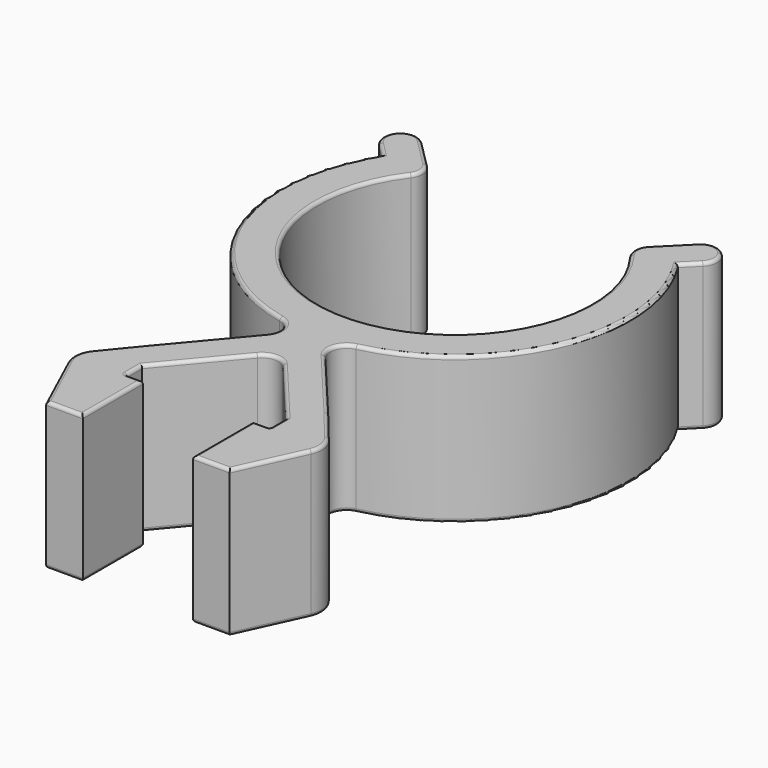
from build123d import *

# Parameters (mm, degrees)
F1_DEPTH      = 8.8
F2_R          = 0.99999
F3_R          = 0.1
F4_R          = 1
F6_T3_DEPTH   = 5.9978588629
F6_T7_ANGLE   = 100
F6_T10_DEPTH  = 1.6
F6_T14_DEPTH  = 5.9978588629
F6_T18_ANGLE  = 90
F6_T21_DEPTH  = 1.6
F6_T25_DEPTH  = 1.4
F6_T28_ANGLE  = 90
F6_T31_DEPTH  = 5.5
F6_T34_DEPTH  = 1.4
F6_T37_DEPTH  = 3.2
F6_T40_DEPTH  = 5.5
F6_T43_DEPTH  = 6.2023355211
F6_T46_DEPTH  = 3.2
F6_T49_DEPTH  = 3.9268834236
F6_T52_DEPTH  = 6.2023355211
F6_T55_DEPTH  = 5.8449118324
F6_T58_DEPTH  = 3.9268834236
F6_T61_ANGLE  = 117.3981887598
F6_T64_DEPTH  = 5.8449118324
F6_T67_ANGLE  = 112.5286263579
F6_T71_ANGLE  = 117.3981887598
F6_T74_DEPTH  = 1.680236188
F6_S75_R      = 10.5
F6_T76_DEPTH  = 2
F6_T79_ANGLE  = 112.5286263579
F6_T83_ANGLE  = 83.5571716204
F6_T86_DEPTH  = 1.680236188
F6_S87_R      = 10.5
F6_T88_DEPTH  = 2
F6_T91_ANGLE  = 0.0001002781
F6_T94_ANGLE  = 83.5571716204
F6_T97_ANGLE  = 96.4427281016
F6_T100_ANGLE = 0.0001002781
F6_T103_DEPTH = 2.3183400779
F6_T106_ANGLE = 96.4427281016
F6_T109_ANGLE = 81.9369478746
F6_T112_DEPTH = 2.3183400779
F6_T115_ANGLE = 253.8738957492
F6_T118_ANGLE = 81.9369478746
F6_T121_DEPTH = 5.9978588629
F6_T125_ANGLE = 100
F6_T128_DEPTH = 1.6
F6_T132_DEPTH = 5.9978588629
F6_T136_ANGLE = 90
F6_T139_DEPTH = 1.6
F6_T143_DEPTH = 1.4
F6_T146_ANGLE = 90
F6_T149_DEPTH = 5.5
F6_T152_DEPTH = 1.4
F6_T155_DEPTH = 3.2
F6_T158_DEPTH = 5.5
F6_T161_DEPTH = 6.2023355211
F6_T164_DEPTH = 3.2
F6_T167_DEPTH = 3.9268834236
F6_T170_DEPTH = 6.2023355211
F6_T173_DEPTH = 5.8449118324
F6_T176_DEPTH = 3.9268834236
F6_T179_ANGLE = 117.3981887598
F6_T182_DEPTH = 5.8449118324
F6_T185_ANGLE = 112.5286263579
F6_T189_ANGLE = 117.3981887598
F6_T192_DEPTH = 1.680236188
F6_S193_R     = 10.5
F6_T194_DEPTH = 2
F6_T197_ANGLE = 112.5286263579
F6_T201_ANGLE = 83.5571716204
F6_T204_DEPTH = 1.680236188
F6_S205_R     = 10.5
F6_T206_DEPTH = 2
F6_T209_ANGLE = 0.0001002781
F6_T212_ANGLE = 83.5571716204
F6_T215_ANGLE = 96.4427281016
F6_T218_ANGLE = 0.0001002781
F6_T221_DEPTH = 2.3183400779
F6_T224_ANGLE = 96.4427281016
F6_T227_ANGLE = 81.9369478746
F6_T230_DEPTH = 2.3183400779
F6_T233_ANGLE = 253.8738957492
F6_T236_ANGLE = 81.9369478746
F6_T240_DEPTH = 5.9978588629
F6_T244_DEPTH = 1.6
F6_T250_DEPTH = 5.9978588629
F6_T254_DEPTH = 1.6
F6_T260_ANGLE = 112.5286263579
F6_T264_DEPTH = 1.680236188
F6_S265_R     = 10.5
F6_T266_DEPTH = 2
F6_T271_ANGLE = 112.5286263579
F6_T275_DEPTH = 1.680236188
F6_S276_R     = 10.5
F6_T277_DEPTH = 2
F6_T282_DEPTH = 5.9978588629
F6_T286_DEPTH = 1.6
F6_T292_DEPTH = 5.9978588629
F6_T296_DEPTH = 1.6
F6_T302_ANGLE = 112.5286263579
F6_T306_DEPTH = 1.680236188
F6_S307_R     = 10.5
F6_T308_DEPTH = 2
F6_T313_ANGLE = 112.5286263579
F6_T317_DEPTH = 1.680236188
F6_S318_R     = 10.5
F6_T319_DEPTH = 2
F7_T1_DEPTH   = 8.8000000003
F7_T4_ANGLE   = 63.917692294
F7_T6_ANGLE   = 63.917692294
F7_T8_ANGLE   = 63.917692294
F7_T10_ANGLE  = 63.917692294


# Not quite as in the source:
# - a fillet or chamfer that OpenCascade refuses, or shapes differently, is made with other operations: its cross-section is extruded or revolved along the edge and cut away or added
# - a fillet or chamfer is up to 0.001 mm smaller than in the source, because OpenCascade refuses the exact size
# - a feature of the source that left no trace in its solid (it failed there, or was rolled back) is left out


with BuildPart() as f1:
    # F0 (on Top) → F1 (new body)
    with BuildSketch(Plane.XY):
        with BuildLine():
            ThreePointArc((6, 5.589275445), (0, -8.2), (-6, 5.589275445))
            Line((-6, 5.589275445), (-9.0418110175, 8.6310864625))
            ThreePointArc((-9.0418110175, 8.6310864625), (-9.706736329, 7.8758662913), (-10.3087630343, 7.0696113545))
            Line((-10.3087630343, 7.0696113545), (-8.8654004375, 5.6262487577))
            ThreePointArc((-8.8654004375, 5.6262487577), (-9.338258559, -4.8007215171), (-0.5833668689, -10.4837819081))
            Line((-0.5833668689, -10.4837819081), (-5.5, -16.3431971055))
            Line((-5.5, -16.3431971055), (-7.669290062, -18.9960654825))
            Line((-7.669290062, -18.9960654825), (-5.5, -23.7245404482))
            Line((-5.5, -23.7245404482), (-3.3, -23.7245404482))
            Line((-3.3, -23.7245404482), (-3.3, -19.2245404482))
            Line((-3.3, -19.2245404482), (-4.3, -19.2245404482))
            Line((-4.3, -19.2245404482), (-4.3, -18.0245404482))
            Line((-4.3, -18.0245404482), (0, -12.9))
            Line((0, -12.9), (4.3, -18.0245404482))
            Line((4.3, -18.0245404482), (4.3, -19.2245404482))
            Line((4.3, -19.2245404482), (3.3, -19.2245404482))
            Line((3.3, -19.2245404482), (3.3, -23.7245404482))
            Line((3.3, -23.7245404482), (5.5, -23.7245404482))
            Line((5.5, -23.7245404482), (7.669290062, -18.9960654825))
            Line((7.669290062, -18.9960654825), (5.5, -16.3431971055))
            Line((5.5, -16.3431971055), (1.5320888862, -11.6144247806))
            Line((1.5320888862, -11.6144247806), (0.5833668689, -10.4837819081))
            ThreePointArc((0.5833668689, -10.4837819081), (9.338258559, -4.8007215171), (8.8654004375, 5.6262487577))
            Line((8.8654004375, 5.6262487577), (10.3087630343, 7.0696113545))
            ThreePointArc((10.3087630343, 7.0696113545), (9.706736329, 7.8758662913), (9.0418110175, 8.6310864625))
            Line((9.0418110175, 8.6310864625), (6, 5.589275445))
        make_face()
    extrude(amount=F1_DEPTH)

    # F2 (radius 1 in the source; OpenCascade refuses exactly that, so slightly less here)
    f2_edges = [f1.edges().sort_by_distance(p)[0] for p in [
        (6, 5.589275, 4.4),
        (-6, 5.589275, 4.4),
        (-9.041811, 8.631086, 4.4),
        (9.041811, 8.631086, 4.4),
        (10.308763, 7.069611, 4.4),
        (-10.308763, 7.069611, 4.4),
        (0.583367, -10.483782, 4.4),
        (-0.583367, -10.483782, 4.4),
    ]]
    fillet(f2_edges, radius=F2_R)

    # F3
    f3_edges = [f1.edges().sort_by_distance(p)[0] for p in [
        (-4.3, -19.22454, 4.4),
        (4.3, -19.22454, 4.4),
    ]]
    fillet(f3_edges, radius=F3_R)

    # F4
    f4_edges = [f1.edges().sort_by_distance(p)[0] for p in [
        (0, -12.9, 4.4),
    ]]
    fillet(f4_edges, radius=F4_R)

    # F6: fillet of radius 0.2 on 72 edges, made by hand


with BuildPart() as f6_tool1:
    # F6_s2 → F6_t3 (new body)
    with BuildSketch(Plane(origin=(7.11805445, -8.4829669631, 0), x_dir=(0, 0, 1), z_dir=(0.6427876097, -0.7660444431, 0))):
        with BuildLine():
            ThreePointArc((8.6, 8.291960165), (8.7414213562, 8.2333815212), (8.8, 8.091960165))
            Line((8.8, 8.091960165), (8.8, 8.291960165))
            Line((8.8, 8.291960165), (8.6, 8.291960165))
        make_face()
    extrude(amount=F6_T3_DEPTH)

    split(bisect_by=Plane.YZ.offset(4.3), keep=Keep.BOTTOM)


with BuildPart() as f6_tool5:
    # F6_s6 → F6_t7 (revolve)
    with BuildSketch(Plane(origin=(7.11805445, -8.4829669631, 0), x_dir=(0, 0, 1), z_dir=(0.6427876097, -0.7660444431, 0))):
        with BuildLine():
            ThreePointArc((8.6, 8.291960165), (8.7414213562, 8.2333815212), (8.8, 8.091960165))
            Line((8.8, 8.091960165), (8.8, 8.291960165))
            Line((8.8, 8.291960165), (8.6, 8.291960165))
        make_face()
    revolve(axis=Axis((0, -14.4557238269, 8.8), (0, 0, 1)), revolution_arc=F6_T7_ANGLE)


with BuildPart() as f6_tool8:
    # F6_s9 → F6_t10 (new body)
    with BuildSketch(Plane.XZ.offset(17.5245404482)):
        with BuildLine():
            ThreePointArc((4.3, 8.6), (4.3585786438, 8.7414213562), (4.5, 8.8))
            Line((4.5, 8.8), (4.3, 8.8))
            Line((4.3, 8.8), (4.3, 8.6))
        make_face()
    extrude(amount=F6_T10_DEPTH)

    split(bisect_by=Plane(origin=(-6.3520100069, -5.329969254, 0), x_dir=(0, 0, 1), z_dir=(-0.7660444431, -0.6427876097, 0)), keep=Keep.TOP)


with BuildPart() as f6_tool12:
    # F6_s13 → F6_t14 (new body)
    with BuildSketch(Plane(origin=(-10.9734038118, -13.0775934157, 0), x_dir=(0, 0, 1), z_dir=(0.6427876097, 0.7660444431, 0))):
        with BuildLine():
            ThreePointArc((8.6, 8.291960165), (8.7414213562, 8.2333815212), (8.8, 8.091960165))
            Line((8.8, 8.091960165), (8.8, 8.291960165))
            Line((8.8, 8.291960165), (8.6, 8.291960165))
        make_face()
    extrude(amount=F6_T14_DEPTH)

    split(bisect_by=Plane.YZ.offset(-4.3), keep=Keep.TOP)


with BuildPart() as f6_tool16:
    # F6_s17 → F6_t18 (revolve)
    with BuildSketch(Plane.YZ.offset(4.2)):
        with BuildLine():
            ThreePointArc((-19.2245404482, 8.6), (-19.2831190919, 8.7414213562), (-19.4245404482, 8.8))
            Line((-19.4245404482, 8.8), (-19.2245404482, 8.8))
            Line((-19.2245404482, 8.8), (-19.2245404482, 8.6))
        make_face()
    revolve(axis=Axis((4.2, -19.1245404482, 8.8), (0, 0, 1)), revolution_arc=F6_T18_ANGLE)


with BuildPart() as f6_tool19:
    # F6_s20 → F6_t21 (new body)
    with BuildSketch(Plane.XZ.offset(19.1245404482)):
        with BuildLine():
            ThreePointArc((-4.3, 8.6), (-4.3585786438, 8.7414213562), (-4.5, 8.8))
            Line((-4.5, 8.8), (-4.3, 8.8))
            Line((-4.3, 8.8), (-4.3, 8.6))
        make_face()
    extrude(amount=-F6_T21_DEPTH)

    split(bisect_by=Plane(origin=(6.3520100069, -5.329969254, 0), x_dir=(0, 0, 1), z_dir=(0.7660444431, -0.6427876097, 0)), keep=Keep.TOP)


with BuildPart() as f6_tool23:
    # F6_s24 → F6_t25 (new body)
    with BuildSketch(Plane.YZ.offset(4.2)):
        with BuildLine():
            ThreePointArc((-19.2245404482, 8.6), (-19.2831190919, 8.7414213562), (-19.4245404482, 8.8))
            Line((-19.4245404482, 8.8), (-19.2245404482, 8.8))
            Line((-19.2245404482, 8.8), (-19.2245404482, 8.6))
        make_face()
    extrude(amount=-F6_T25_DEPTH)


with BuildPart() as f6_tool26:
    # F6_s27 → F6_t28 (revolve)
    with BuildSketch(Plane.YZ.offset(-4.2)):
        with BuildLine():
            ThreePointArc((-19.2245404482, 8.6), (-19.2831190919, 8.7414213562), (-19.4245404482, 8.8))
            Line((-19.4245404482, 8.8), (-19.2245404482, 8.8))
            Line((-19.2245404482, 8.8), (-19.2245404482, 8.6))
        make_face()
    revolve(axis=Axis((-4.2, -19.1245404482, 8.8), (0, 0, -1)), revolution_arc=F6_T28_ANGLE)


with BuildPart() as f6_tool29:
    # F6_s30 → F6_t31 (new body)
    with BuildSketch(Plane.XZ.offset(18.7245404482)):
        with BuildLine():
            ThreePointArc((3.3, 8.6), (3.3585786438, 8.7414213562), (3.5, 8.8))
            Line((3.5, 8.8), (3.3, 8.8))
            Line((3.3, 8.8), (3.3, 8.6))
        make_face()
    extrude(amount=F6_T31_DEPTH)


with BuildPart() as f6_tool32:
    # F6_s33 → F6_t34 (new body)
    with BuildSketch(Plane.YZ.offset(-2.8)):
        with BuildLine():
            ThreePointArc((-19.2245404482, 8.6), (-19.2831190919, 8.7414213562), (-19.4245404482, 8.8))
            Line((-19.4245404482, 8.8), (-19.2245404482, 8.8))
            Line((-19.2245404482, 8.8), (-19.2245404482, 8.6))
        make_face()
    extrude(amount=-F6_T34_DEPTH)


with BuildPart() as f6_tool35:
    # F6_s36 → F6_t37 (new body)
    with BuildSketch(Plane.YZ.offset(2.8)):
        with BuildLine():
            ThreePointArc((-23.7245404482, 8.6), (-23.6659618044, 8.7414213562), (-23.5245404482, 8.8))
            Line((-23.5245404482, 8.8), (-23.7245404482, 8.8))
            Line((-23.7245404482, 8.8), (-23.7245404482, 8.6))
        make_face()
    extrude(amount=F6_T37_DEPTH)


with BuildPart() as f6_tool38:
    # F6_s39 → F6_t40 (new body)
    with BuildSketch(Plane.XZ.offset(24.2245404482)):
        with BuildLine():
            ThreePointArc((-3.3, 8.6), (-3.3585786438, 8.7414213562), (-3.5, 8.8))
            Line((-3.5, 8.8), (-3.3, 8.8))
            Line((-3.3, 8.8), (-3.3, 8.6))
        make_face()
    extrude(amount=-F6_T40_DEPTH)


with BuildPart() as f6_tool41:
    # F6_s42 → F6_t43 (new body)
    with BuildSketch(Plane(origin=(-8.2438350525, -17.9693662682, 0), x_dir=(0, 0, 1), z_dir=(0.4169838822, 0.9089138804, 0))):
        with BuildLine():
            ThreePointArc((8.6, 14.8917773215), (8.7414213562, 14.8331986777), (8.8, 14.6917773215))
            Line((8.8, 14.6917773215), (8.8, 14.8917773215))
            Line((8.8, 14.8917773215), (8.6, 14.8917773215))
        make_face()
    extrude(amount=F6_T43_DEPTH)


with BuildPart() as f6_tool44:
    # F6_s45 → F6_t46 (new body)
    with BuildSketch(Plane.YZ.offset(-6)):
        with BuildLine():
            ThreePointArc((-23.7245404482, 8.6), (-23.6659618044, 8.7414213562), (-23.5245404482, 8.8))
            Line((-23.5245404482, 8.8), (-23.7245404482, 8.8))
            Line((-23.7245404482, 8.8), (-23.7245404482, 8.6))
        make_face()
    extrude(amount=F6_T46_DEPTH)


with BuildPart() as f6_tool47:
    # F6_s48 → F6_t49 (new body)
    with BuildSketch(Plane(origin=(12.6986163819, -15.5293929659, 0), x_dir=(0, 0, 1), z_dir=(-0.6330212598, 0.7741344099, 0))):
        with BuildLine():
            ThreePointArc((8.6, -6.0878519667), (8.7414213562, -6.1464306105), (8.8, -6.2878519667))
            Line((8.8, -6.2878519667), (8.8, -6.0878519667))
            Line((8.8, -6.0878519667), (8.6, -6.0878519667))
        make_face()
    extrude(amount=F6_T49_DEPTH)


with BuildPart() as f6_tool50:
    # F6_s51 → F6_t52 (new body)
    with BuildSketch(Plane(origin=(5.6575611083, -12.3319774221, 0), x_dir=(0, 0, 1), z_dir=(0.4169838822, -0.9089138804, 0))):
        with BuildLine():
            ThreePointArc((8.6, 14.8917773215), (8.7414213562, 14.8331986777), (8.8, 14.6917773215))
            Line((8.8, 14.6917773215), (8.8, 14.8917773215))
            Line((8.8, 14.8917773215), (8.6, 14.8917773215))
        make_face()
    extrude(amount=F6_T52_DEPTH)


with BuildPart() as f6_tool53:
    # F6_s54 → F6_t55 (new body)
    with BuildSketch(Plane(origin=(6.5628842151, -7.8213408411, 0), x_dir=(0, 0, 1), z_dir=(0.6427876097, -0.7660444431, 0))):
        with BuildLine():
            ThreePointArc((8.6, 6.291960165), (8.7414213562, 6.3505388087), (8.8, 6.491960165))
            Line((8.8, 6.491960165), (8.8, 6.291960165))
            Line((8.8, 6.291960165), (8.6, 6.291960165))
        make_face()
    extrude(amount=F6_T55_DEPTH)


with BuildPart() as f6_tool56:
    # F6_s57 → F6_t58 (new body)
    with BuildSketch(Plane(origin=(-10.2128156899, -12.489457384, 0), x_dir=(0, 0, 1), z_dir=(-0.6330212598, -0.7741344099, 0))):
        with BuildLine():
            ThreePointArc((8.6, -6.0878519667), (8.7414213562, -6.1464306105), (8.8, -6.2878519667))
            Line((8.8, -6.2878519667), (8.8, -6.0878519667))
            Line((8.8, -6.0878519667), (8.6, -6.0878519667))
        make_face()
    extrude(amount=F6_T58_DEPTH)


with BuildPart() as f6_tool59:
    # F6_s60 → F6_t61 (revolve)
    with BuildSketch(Plane(origin=(0, 0, 0), x_dir=(0, 0, 1), z_dir=(0.9759098655, 0.2181740921, 0))):
        with BuildLine():
            ThreePointArc((8.6, 10.5), (8.7414213562, 10.4414213562), (8.8, 10.3))
            Line((8.8, 10.3), (8.8, 10.5))
            Line((8.8, 10.5), (8.6, 10.5))
        make_face()
    revolve(axis=Axis((2.5089998771, -11.222953694, 8.8), (0, 0, 1)), revolution_arc=F6_T61_ANGLE)


with BuildPart() as f6_tool62:
    # F6_s63 → F6_t64 (new body)
    with BuildSketch(Plane(origin=(-6.5628842151, -7.8213408411, 0), x_dir=(0, 0, 1), z_dir=(-0.6427876097, -0.7660444431, 0))):
        with BuildLine():
            ThreePointArc((8.6, -6.291960165), (8.7414213562, -6.3505388087), (8.8, -6.491960165))
            Line((8.8, -6.491960165), (8.8, -6.291960165))
            Line((8.8, -6.291960165), (8.6, -6.291960165))
        make_face()
    extrude(amount=F6_T64_DEPTH)


with BuildPart() as f6_tool65:
    # F6_s66 → F6_t67 (revolve)
    with BuildSketch(Plane(origin=(0, 0, 0), x_dir=(0, 0, 1), z_dir=(-0.9759098655, -0.2181740921, 0))):
        with BuildLine():
            ThreePointArc((8.6, -10.5), (8.7414213562, -10.4414213562), (8.8, -10.3))
            Line((8.8, -10.3), (8.8, -10.5))
            Line((8.8, -10.5), (8.6, -10.5))
        make_face()
    revolve(axis=Axis((0, 0, 8.8), (0, 0, 1)), revolution_arc=F6_T67_ANGLE)

    split(bisect_by=Plane(origin=(1.6195758399, -1.6195758399, 0), x_dir=(0, 0, 1), z_dir=(0.7071067812, -0.7071067812, 0)), keep=Keep.TOP)


with BuildPart() as f6_tool69:
    # F6_s70 → F6_t71 (revolve)
    with BuildSketch(Plane(origin=(-6.5628842151, -7.8213408411, 0), x_dir=(0, 0, 1), z_dir=(-0.6427876097, -0.7660444431, 0))):
        with BuildLine():
            ThreePointArc((8.6, -6.291960165), (8.7414213562, -6.3505388087), (8.8, -6.491960165))
            Line((8.8, -6.491960165), (8.8, -6.291960165))
            Line((8.8, -6.291960165), (8.6, -6.291960165))
        make_face()
    revolve(axis=Axis((-2.5089998771, -11.222953694, 8.8), (0, 0, 1)), revolution_arc=F6_T71_ANGLE)


with BuildPart() as f6_tool72:
    # F6_s73 → F6_t74 (new body)
    with BuildSketch(Plane(origin=(6.892271207, 6.892271207, 0), x_dir=(0, 0, 1), z_dir=(0.7071067812, 0.7071067812, 0))):
        with BuildLine():
            ThreePointArc((8.6, 2.290426118), (8.7414213562, 2.2318474743), (8.8, 2.090426118))
            Line((8.8, 2.090426118), (8.8, 2.290426118))
            Line((8.8, 2.290426118), (8.6, 2.290426118))
        make_face()
    extrude(amount=F6_T74_DEPTH)

    # F6_s75 → F6_t76 (cut, symmetric)
    with BuildSketch(Plane.XY.offset(8.7)):
        Circle(F6_S75_R)
    extrude(amount=F6_T76_DEPTH, both=True, mode=Mode.SUBTRACT)


with BuildPart() as f6_tool77:
    # F6_s78 → F6_t79 (revolve)
    with BuildSketch(Plane(origin=(0, 0, 0), x_dir=(0, 0, 1), z_dir=(0.5754398017, 0.8178441383, 0))):
        with BuildLine():
            ThreePointArc((8.6, -10.5), (8.7414213562, -10.4414213562), (8.8, -10.3))
            Line((8.8, -10.3), (8.8, -10.5))
            Line((8.8, -10.5), (8.6, -10.5))
        make_face()
    revolve(axis=Axis((0, 0, 8.8), (0, 0, 1)), revolution_arc=F6_T79_ANGLE)

    split(bisect_by=Plane(origin=(-1.6195758399, -1.6195758399, 0), x_dir=(0, 0, 1), z_dir=(-0.7071067812, -0.7071067812, 0)), keep=Keep.TOP)


with BuildPart() as f6_tool81:
    # F6_s82 → F6_t83 (revolve)
    with BuildSketch(Plane(origin=(0, 0, 0), x_dir=(0, 0, 1), z_dir=(-0.6232952389, 0.7819866017, 0))):
        with BuildLine():
            ThreePointArc((8.6, 12.5), (8.7414213562, 12.4414213562), (8.8, 12.3))
            Line((8.8, 12.3), (8.8, 12.5))
            Line((8.8, 12.5), (8.6, 12.5))
        make_face()
    revolve(axis=Axis((8.9928537393, 7.1679014798, 8.8), (0, 0, -1)), revolution_arc=F6_T83_ANGLE)


with BuildPart() as f6_tool84:
    # F6_s85 → F6_t86 (new body)
    with BuildSketch(Plane(origin=(-8.0803776095, 8.0803776095, 0), x_dir=(0, 0, 1), z_dir=(0.7071067812, -0.7071067812, 0))):
        with BuildLine():
            ThreePointArc((8.6, 2.290426118), (8.7414213562, 2.2318474743), (8.8, 2.090426118))
            Line((8.8, 2.090426118), (8.8, 2.290426118))
            Line((8.8, 2.290426118), (8.6, 2.290426118))
        make_face()
    extrude(amount=F6_T86_DEPTH)

    # F6_s87 → F6_t88 (cut, symmetric)
    with BuildSketch(Plane.XY.offset(8.7)):
        Circle(F6_S87_R)
    extrude(amount=F6_T88_DEPTH, both=True, mode=Mode.SUBTRACT)


with BuildPart() as f6_tool89:
    # F6_s90 → F6_t91 (revolve)
    with BuildSketch(Plane(origin=(0, 0, 0), x_dir=(0, 0, 1), z_dir=(0.6232952389, -0.7819866017, 0))):
        with BuildLine():
            ThreePointArc((8.6, -12.5), (8.7414213562, -12.4414213562), (8.8, -12.3))
            Line((8.8, -12.3), (8.8, -12.5))
            Line((8.8, -12.5), (8.6, -12.5))
        make_face()
    revolve(axis=Axis((0, 0, 8.8), (0, 0, 1)), revolution_arc=F6_T91_ANGLE)


with BuildPart() as f6_tool92:
    # F6_s93 → F6_t94 (revolve)
    with BuildSketch(Plane(origin=(-8.0803776095, 8.0803776095, 0), x_dir=(0, 0, 1), z_dir=(0.7071067812, -0.7071067812, 0))):
        with BuildLine():
            ThreePointArc((8.6, 2.290426118), (8.7414213562, 2.2318474743), (8.8, 2.090426118))
            Line((8.8, 2.090426118), (8.8, 2.290426118))
            Line((8.8, 2.290426118), (8.6, 2.290426118))
        make_face()
    revolve(axis=Axis((-8.9928537393, 7.1679014798, 8.8), (0, 0, -1)), revolution_arc=F6_T94_ANGLE)


with BuildPart() as f6_tool95:
    # F6_s96 → F6_t97 (revolve)
    with BuildSketch(Plane(origin=(0, 0, 0), x_dir=(0, 0, 1), z_dir=(0.6232966075, -0.7819855108, 0))):
        with BuildLine():
            ThreePointArc((8.6, -12.5), (8.7414213562, -12.4414213562), (8.8, -12.3))
            Line((8.8, -12.3), (8.8, -12.5))
            Line((8.8, -12.5), (8.6, -12.5))
        make_face()
    revolve(axis=Axis((8.9928411941, 7.1679172189, 8.8), (0, 0, 1)), revolution_arc=F6_T97_ANGLE)


with BuildPart() as f6_tool98:
    # F6_s99 → F6_t100 (revolve)
    with BuildSketch(Plane(origin=(0, 0, 0), x_dir=(0, 0, 1), z_dir=(0.6232966075, 0.7819855108, 0))):
        with BuildLine():
            ThreePointArc((8.6, -12.5), (8.7414213562, -12.4414213562), (8.8, -12.3))
            Line((8.8, -12.3), (8.8, -12.5))
            Line((8.8, -12.5), (8.6, -12.5))
        make_face()
    revolve(axis=Axis((0, 0, 8.8), (0, 0, 1)), revolution_arc=F6_T100_ANGLE)


with BuildPart() as f6_tool101:
    # F6_s102 → F6_t103 (new body)
    with BuildSketch(Plane(origin=(8.0803792065, 8.0803792065, 0), x_dir=(0, 0, 1), z_dir=(-0.7071067812, -0.7071067812, 0))):
        with BuildLine():
            ThreePointArc((8.6, -0.290426118), (8.7414213562, -0.3490047618), (8.8, -0.490426118))
            Line((8.8, -0.490426118), (8.8, -0.290426118))
            Line((8.8, -0.290426118), (8.6, -0.290426118))
        make_face()
    extrude(amount=F6_T103_DEPTH)


with BuildPart() as f6_tool104:
    # F6_s105 → F6_t106 (revolve)
    with BuildSketch(Plane(origin=(0, 0, 0), x_dir=(0, 0, 1), z_dir=(-0.6232966075, -0.7819855108, 0))):
        with BuildLine():
            ThreePointArc((8.6, 12.5), (8.7414213562, 12.4414213562), (8.8, 12.3))
            Line((8.8, 12.3), (8.8, 12.5))
            Line((8.8, 12.5), (8.6, 12.5))
        make_face()
    revolve(axis=Axis((-8.9928411941, 7.1679172189, 8.8), (0, 0, -1)), revolution_arc=F6_T106_ANGLE)


with BuildPart() as f6_tool107:
    # F6_s108 → F6_t109 (revolve)
    with BuildSketch(Plane(origin=(0, 0, 0), x_dir=(0, 0, 1), z_dir=(0.6009357867, -0.799297304, 0))):
        with BuildLine():
            ThreePointArc((8.6, -8.2), (8.7414213562, -8.2585786438), (8.8, -8.4))
            Line((8.8, -8.4), (8.8, -8.2))
            Line((8.8, -8.2), (8.6, -8.2))
        make_face()
    revolve(axis=Axis((7.353527204, 5.5286032287, 8.8), (0, 0, -1)), revolution_arc=F6_T109_ANGLE)


with BuildPart() as f6_tool110:
    # F6_s111 → F6_t112 (new body)
    with BuildSketch(Plane(origin=(-6.4410652163, 6.4410652163, 0), x_dir=(0, 0, 1), z_dir=(-0.7071067812, 0.7071067812, 0))):
        with BuildLine():
            ThreePointArc((8.6, -0.290426118), (8.7414213562, -0.3490047618), (8.8, -0.490426118))
            Line((8.8, -0.490426118), (8.8, -0.290426118))
            Line((8.8, -0.290426118), (8.6, -0.290426118))
        make_face()
    extrude(amount=F6_T112_DEPTH)


with BuildPart() as f6_tool113:
    # F6_s114 → F6_t115 (revolve)
    with BuildSketch(Plane(origin=(0, 0, 0), x_dir=(0, 0, 1), z_dir=(-0.6009357867, 0.799297304, 0))):
        with BuildLine():
            ThreePointArc((8.6, 8.2), (8.7414213562, 8.2585786438), (8.8, 8.4))
            Line((8.8, 8.4), (8.8, 8.2))
            Line((8.8, 8.2), (8.6, 8.2))
        make_face()
    revolve(axis=Axis((0, 0, 8.8), (0, 0, -1)), revolution_arc=F6_T115_ANGLE)


with BuildPart() as f6_tool116:
    # F6_s117 → F6_t118 (revolve)
    with BuildSketch(Plane(origin=(0, 0, 0), x_dir=(0, 0, 1), z_dir=(-0.6009357867, -0.799297304, 0))):
        with BuildLine():
            ThreePointArc((8.6, 8.2), (8.7414213562, 8.2585786438), (8.8, 8.4))
            Line((8.8, 8.4), (8.8, 8.2))
            Line((8.8, 8.2), (8.6, 8.2))
        make_face()
    revolve(axis=Axis((-7.353527204, 5.5286032287, 8.8), (0, 0, 1)), revolution_arc=F6_T118_ANGLE)


with BuildPart() as f6_tool119:
    # F6_s120 → F6_t121 (new body)
    with BuildSketch(Plane(origin=(7.11805445, -8.4829669631, 0), x_dir=(0, 0, 1), z_dir=(0.6427876097, -0.7660444431, 0))):
        with BuildLine():
            ThreePointArc((0, 8.091960165), (0.0585786438, 8.2333815212), (0.2, 8.291960165))
            Line((0.2, 8.291960165), (0, 8.291960165))
            Line((0, 8.291960165), (0, 8.091960165))
        make_face()
    extrude(amount=F6_T121_DEPTH)

    split(bisect_by=Plane.YZ.offset(4.3), keep=Keep.BOTTOM)


with BuildPart() as f6_tool123:
    # F6_s124 → F6_t125 (revolve)
    with BuildSketch(Plane(origin=(7.11805445, -8.4829669631, 0), x_dir=(0, 0, 1), z_dir=(0.6427876097, -0.7660444431, 0))):
        with BuildLine():
            ThreePointArc((0, 8.091960165), (0.0585786438, 8.2333815212), (0.2, 8.291960165))
            Line((0.2, 8.291960165), (0, 8.291960165))
            Line((0, 8.291960165), (0, 8.091960165))
        make_face()
    revolve(axis=Axis((0, -14.4557238269, 0), (0, 0, 1)), revolution_arc=F6_T125_ANGLE)


with BuildPart() as f6_tool126:
    # F6_s127 → F6_t128 (new body)
    with BuildSketch(Plane.XZ.offset(17.5245404482)):
        with BuildLine():
            ThreePointArc((4.5, 0), (4.3585786438, 0.0585786438), (4.3, 0.2))
            Line((4.3, 0.2), (4.3, 0))
            Line((4.3, 0), (4.5, 0))
        make_face()
    extrude(amount=F6_T128_DEPTH)

    split(bisect_by=Plane(origin=(-6.3520100069, -5.329969254, 0), x_dir=(0, 0, 1), z_dir=(-0.7660444431, -0.6427876097, 0)), keep=Keep.TOP)


with BuildPart() as f6_tool130:
    # F6_s131 → F6_t132 (new body)
    with BuildSketch(Plane(origin=(-10.9734038118, -13.0775934157, 0), x_dir=(0, 0, 1), z_dir=(0.6427876097, 0.7660444431, 0))):
        with BuildLine():
            ThreePointArc((0, 8.091960165), (0.0585786438, 8.2333815212), (0.2, 8.291960165))
            Line((0.2, 8.291960165), (0, 8.291960165))
            Line((0, 8.291960165), (0, 8.091960165))
        make_face()
    extrude(amount=F6_T132_DEPTH)

    split(bisect_by=Plane.YZ.offset(-4.3), keep=Keep.TOP)


with BuildPart() as f6_tool134:
    # F6_s135 → F6_t136 (revolve)
    with BuildSketch(Plane.YZ.offset(4.2)):
        with BuildLine():
            ThreePointArc((-19.4245404482, 0), (-19.2831190919, 0.0585786438), (-19.2245404482, 0.2))
            Line((-19.2245404482, 0.2), (-19.2245404482, 0))
            Line((-19.2245404482, 0), (-19.4245404482, 0))
        make_face()
    revolve(axis=Axis((4.2, -19.1245404482, 0), (0, 0, 1)), revolution_arc=F6_T136_ANGLE)


with BuildPart() as f6_tool137:
    # F6_s138 → F6_t139 (new body)
    with BuildSketch(Plane.XZ.offset(19.1245404482)):
        with BuildLine():
            ThreePointArc((-4.5, 0), (-4.3585786438, 0.0585786438), (-4.3, 0.2))
            Line((-4.3, 0.2), (-4.3, 0))
            Line((-4.3, 0), (-4.5, 0))
        make_face()
    extrude(amount=-F6_T139_DEPTH)

    split(bisect_by=Plane(origin=(6.3520100069, -5.329969254, 0), x_dir=(0, 0, 1), z_dir=(0.7660444431, -0.6427876097, 0)), keep=Keep.TOP)


with BuildPart() as f6_tool141:
    # F6_s142 → F6_t143 (new body)
    with BuildSketch(Plane.YZ.offset(4.2)):
        with BuildLine():
            ThreePointArc((-19.4245404482, 0), (-19.2831190919, 0.0585786438), (-19.2245404482, 0.2))
            Line((-19.2245404482, 0.2), (-19.2245404482, 0))
            Line((-19.2245404482, 0), (-19.4245404482, 0))
        make_face()
    extrude(amount=-F6_T143_DEPTH)


with BuildPart() as f6_tool144:
    # F6_s145 → F6_t146 (revolve)
    with BuildSketch(Plane.YZ.offset(-4.2)):
        with BuildLine():
            ThreePointArc((-19.4245404482, 0), (-19.2831190919, 0.0585786438), (-19.2245404482, 0.2))
            Line((-19.2245404482, 0.2), (-19.2245404482, 0))
            Line((-19.2245404482, 0), (-19.4245404482, 0))
        make_face()
    revolve(axis=Axis((-4.2, -19.1245404482, 0), (0, 0, -1)), revolution_arc=F6_T146_ANGLE)


with BuildPart() as f6_tool147:
    # F6_s148 → F6_t149 (new body)
    with BuildSketch(Plane.XZ.offset(18.7245404482)):
        with BuildLine():
            ThreePointArc((3.5, 0), (3.3585786438, 0.0585786438), (3.3, 0.2))
            Line((3.3, 0.2), (3.3, 0))
            Line((3.3, 0), (3.5, 0))
        make_face()
    extrude(amount=F6_T149_DEPTH)


with BuildPart() as f6_tool150:
    # F6_s151 → F6_t152 (new body)
    with BuildSketch(Plane.YZ.offset(-2.8)):
        with BuildLine():
            ThreePointArc((-19.4245404482, 0), (-19.2831190919, 0.0585786438), (-19.2245404482, 0.2))
            Line((-19.2245404482, 0.2), (-19.2245404482, 0))
            Line((-19.2245404482, 0), (-19.4245404482, 0))
        make_face()
    extrude(amount=-F6_T152_DEPTH)


with BuildPart() as f6_tool153:
    # F6_s154 → F6_t155 (new body)
    with BuildSketch(Plane.YZ.offset(2.8)):
        with BuildLine():
            ThreePointArc((-23.5245404482, 0), (-23.6659618044, 0.0585786438), (-23.7245404482, 0.2))
            Line((-23.7245404482, 0.2), (-23.7245404482, 0))
            Line((-23.7245404482, 0), (-23.5245404482, 0))
        make_face()
    extrude(amount=F6_T155_DEPTH)


with BuildPart() as f6_tool156:
    # F6_s157 → F6_t158 (new body)
    with BuildSketch(Plane.XZ.offset(24.2245404482)):
        with BuildLine():
            ThreePointArc((-3.5, 0), (-3.3585786438, 0.0585786438), (-3.3, 0.2))
            Line((-3.3, 0.2), (-3.3, 0))
            Line((-3.3, 0), (-3.5, 0))
        make_face()
    extrude(amount=-F6_T158_DEPTH)


with BuildPart() as f6_tool159:
    # F6_s160 → F6_t161 (new body)
    with BuildSketch(Plane(origin=(-8.2438350525, -17.9693662682, 0), x_dir=(0, 0, 1), z_dir=(0.4169838822, 0.9089138804, 0))):
        with BuildLine():
            ThreePointArc((0, 14.6917773215), (0.0585786438, 14.8331986777), (0.2, 14.8917773215))
            Line((0.2, 14.8917773215), (0, 14.8917773215))
            Line((0, 14.8917773215), (0, 14.6917773215))
        make_face()
    extrude(amount=F6_T161_DEPTH)


with BuildPart() as f6_tool162:
    # F6_s163 → F6_t164 (new body)
    with BuildSketch(Plane.YZ.offset(-6)):
        with BuildLine():
            ThreePointArc((-23.5245404482, 0), (-23.6659618044, 0.0585786438), (-23.7245404482, 0.2))
            Line((-23.7245404482, 0.2), (-23.7245404482, 0))
            Line((-23.7245404482, 0), (-23.5245404482, 0))
        make_face()
    extrude(amount=F6_T164_DEPTH)


with BuildPart() as f6_tool165:
    # F6_s166 → F6_t167 (new body)
    with BuildSketch(Plane(origin=(12.6986163819, -15.5293929659, 0), x_dir=(0, 0, 1), z_dir=(-0.6330212598, 0.7741344099, 0))):
        with BuildLine():
            ThreePointArc((0, -6.2878519667), (0.0585786438, -6.1464306105), (0.2, -6.0878519667))
            Line((0.2, -6.0878519667), (0, -6.0878519667))
            Line((0, -6.0878519667), (0, -6.2878519667))
        make_face()
    extrude(amount=F6_T167_DEPTH)


with BuildPart() as f6_tool168:
    # F6_s169 → F6_t170 (new body)
    with BuildSketch(Plane(origin=(5.6575611083, -12.3319774221, 0), x_dir=(0, 0, 1), z_dir=(0.4169838822, -0.9089138804, 0))):
        with BuildLine():
            ThreePointArc((0, 14.6917773215), (0.0585786438, 14.8331986777), (0.2, 14.8917773215))
            Line((0.2, 14.8917773215), (0, 14.8917773215))
            Line((0, 14.8917773215), (0, 14.6917773215))
        make_face()
    extrude(amount=F6_T170_DEPTH)


with BuildPart() as f6_tool171:
    # F6_s172 → F6_t173 (new body)
    with BuildSketch(Plane(origin=(10.3199211207, -12.2988030709, 0), x_dir=(0, 0, 1), z_dir=(-0.6427876097, 0.7660444431, 0))):
        with BuildLine():
            ThreePointArc((0, -6.491960165), (0.0585786438, -6.3505388087), (0.2, -6.291960165))
            Line((0.2, -6.291960165), (0, -6.291960165))
            Line((0, -6.291960165), (0, -6.491960165))
        make_face()
    extrude(amount=F6_T173_DEPTH)


with BuildPart() as f6_tool174:
    # F6_s175 → F6_t176 (new body)
    with BuildSketch(Plane(origin=(-10.2128156899, -12.489457384, 0), x_dir=(0, 0, 1), z_dir=(-0.6330212598, -0.7741344099, 0))):
        with BuildLine():
            ThreePointArc((0, -6.2878519667), (0.0585786438, -6.1464306105), (0.2, -6.0878519667))
            Line((0.2, -6.0878519667), (0, -6.0878519667))
            Line((0, -6.0878519667), (0, -6.2878519667))
        make_face()
    extrude(amount=F6_T176_DEPTH)


with BuildPart() as f6_tool177:
    # F6_s178 → F6_t179 (revolve)
    with BuildSketch(Plane(origin=(0, 0, 0), x_dir=(0, 0, 1), z_dir=(0.9759098655, 0.2181740921, 0))):
        with BuildLine():
            ThreePointArc((0, 10.3), (0.0585786438, 10.4414213562), (0.2, 10.5))
            Line((0.2, 10.5), (0, 10.5))
            Line((0, 10.5), (0, 10.3))
        make_face()
    revolve(axis=Axis((2.5089998771, -11.222953694, 0), (0, 0, 1)), revolution_arc=F6_T179_ANGLE)


with BuildPart() as f6_tool180:
    # F6_s181 → F6_t182 (new body)
    with BuildSketch(Plane(origin=(-6.5628842151, -7.8213408411, 0), x_dir=(0, 0, 1), z_dir=(-0.6427876097, -0.7660444431, 0))):
        with BuildLine():
            ThreePointArc((0, -6.491960165), (0.0585786438, -6.3505388087), (0.2, -6.291960165))
            Line((0.2, -6.291960165), (0, -6.291960165))
            Line((0, -6.291960165), (0, -6.491960165))
        make_face()
    extrude(amount=F6_T182_DEPTH)


with BuildPart() as f6_tool183:
    # F6_s184 → F6_t185 (revolve)
    with BuildSketch(Plane(origin=(0, 0, 0), x_dir=(0, 0, 1), z_dir=(-0.9759098655, -0.2181740921, 0))):
        with BuildLine():
            ThreePointArc((0, -10.3), (0.0585786438, -10.4414213562), (0.2, -10.5))
            Line((0.2, -10.5), (0, -10.5))
            Line((0, -10.5), (0, -10.3))
        make_face()
    revolve(axis=Axis((0, 0, 0), (0, 0, 1)), revolution_arc=F6_T185_ANGLE)

    split(bisect_by=Plane(origin=(1.6195758399, -1.6195758399, 0), x_dir=(0, 0, 1), z_dir=(0.7071067812, -0.7071067812, 0)), keep=Keep.TOP)


with BuildPart() as f6_tool187:
    # F6_s188 → F6_t189 (revolve)
    with BuildSketch(Plane(origin=(-6.5628842151, -7.8213408411, 0), x_dir=(0, 0, 1), z_dir=(-0.6427876097, -0.7660444431, 0))):
        with BuildLine():
            ThreePointArc((0, -6.491960165), (0.0585786438, -6.3505388087), (0.2, -6.291960165))
            Line((0.2, -6.291960165), (0, -6.291960165))
            Line((0, -6.291960165), (0, -6.491960165))
        make_face()
    revolve(axis=Axis((-2.5089998771, -11.222953694, 0), (0, 0, 1)), revolution_arc=F6_T189_ANGLE)


with BuildPart() as f6_tool190:
    # F6_s191 → F6_t192 (new body)
    with BuildSketch(Plane(origin=(6.892271207, 6.892271207, 0), x_dir=(0, 0, 1), z_dir=(0.7071067812, 0.7071067812, 0))):
        with BuildLine():
            ThreePointArc((0, 2.090426118), (0.0585786438, 2.2318474743), (0.2, 2.290426118))
            Line((0.2, 2.290426118), (0, 2.290426118))
            Line((0, 2.290426118), (0, 2.090426118))
        make_face()
    extrude(amount=F6_T192_DEPTH)

    # F6_s193 → F6_t194 (cut, symmetric)
    with BuildSketch(Plane.XY.offset(0.1)):
        Circle(F6_S193_R)
    extrude(amount=F6_T194_DEPTH, both=True, mode=Mode.SUBTRACT)


with BuildPart() as f6_tool195:
    # F6_s196 → F6_t197 (revolve)
    with BuildSketch(Plane(origin=(0, 0, 0), x_dir=(0, 0, 1), z_dir=(0.5754398017, 0.8178441383, 0))):
        with BuildLine():
            ThreePointArc((0, -10.3), (0.0585786438, -10.4414213562), (0.2, -10.5))
            Line((0.2, -10.5), (0, -10.5))
            Line((0, -10.5), (0, -10.3))
        make_face()
    revolve(axis=Axis((0, 0, 0), (0, 0, 1)), revolution_arc=F6_T197_ANGLE)

    split(bisect_by=Plane(origin=(-1.6195758399, -1.6195758399, 0), x_dir=(0, 0, 1), z_dir=(-0.7071067812, -0.7071067812, 0)), keep=Keep.TOP)


with BuildPart() as f6_tool199:
    # F6_s200 → F6_t201 (revolve)
    with BuildSketch(Plane(origin=(0, 0, 0), x_dir=(0, 0, 1), z_dir=(-0.6232952389, 0.7819866017, 0))):
        with BuildLine():
            ThreePointArc((0, 12.3), (0.0585786438, 12.4414213562), (0.2, 12.5))
            Line((0.2, 12.5), (0, 12.5))
            Line((0, 12.5), (0, 12.3))
        make_face()
    revolve(axis=Axis((8.9928537393, 7.1679014798, 0), (0, 0, -1)), revolution_arc=F6_T201_ANGLE)


with BuildPart() as f6_tool202:
    # F6_s203 → F6_t204 (new body)
    with BuildSketch(Plane(origin=(-8.0803776095, 8.0803776095, 0), x_dir=(0, 0, 1), z_dir=(0.7071067812, -0.7071067812, 0))):
        with BuildLine():
            ThreePointArc((0, 2.090426118), (0.0585786438, 2.2318474743), (0.2, 2.290426118))
            Line((0.2, 2.290426118), (0, 2.290426118))
            Line((0, 2.290426118), (0, 2.090426118))
        make_face()
    extrude(amount=F6_T204_DEPTH)

    # F6_s205 → F6_t206 (cut, symmetric)
    with BuildSketch(Plane.XY.offset(0.1)):
        Circle(F6_S205_R)
    extrude(amount=F6_T206_DEPTH, both=True, mode=Mode.SUBTRACT)


with BuildPart() as f6_tool207:
    # F6_s208 → F6_t209 (revolve)
    with BuildSketch(Plane(origin=(0, 0, 0), x_dir=(0, 0, 1), z_dir=(0.6232952389, -0.7819866017, 0))):
        with BuildLine():
            ThreePointArc((0, -12.3), (0.0585786438, -12.4414213562), (0.2, -12.5))
            Line((0.2, -12.5), (0, -12.5))
            Line((0, -12.5), (0, -12.3))
        make_face()
    revolve(axis=Axis((0, 0, 0), (0, 0, 1)), revolution_arc=F6_T209_ANGLE)


with BuildPart() as f6_tool210:
    # F6_s211 → F6_t212 (revolve)
    with BuildSketch(Plane(origin=(-8.0803776095, 8.0803776095, 0), x_dir=(0, 0, 1), z_dir=(0.7071067812, -0.7071067812, 0))):
        with BuildLine():
            ThreePointArc((0, 2.090426118), (0.0585786438, 2.2318474743), (0.2, 2.290426118))
            Line((0.2, 2.290426118), (0, 2.290426118))
            Line((0, 2.290426118), (0, 2.090426118))
        make_face()
    revolve(axis=Axis((-8.9928537393, 7.1679014798, 0), (0, 0, -1)), revolution_arc=F6_T212_ANGLE)


with BuildPart() as f6_tool213:
    # F6_s214 → F6_t215 (revolve)
    with BuildSketch(Plane(origin=(0, 0, 0), x_dir=(0, 0, 1), z_dir=(0.6232966075, -0.7819855108, 0))):
        with BuildLine():
            ThreePointArc((0, -12.3), (0.0585786438, -12.4414213562), (0.2, -12.5))
            Line((0.2, -12.5), (0, -12.5))
            Line((0, -12.5), (0, -12.3))
        make_face()
    revolve(axis=Axis((8.9928411941, 7.1679172189, 0), (0, 0, 1)), revolution_arc=F6_T215_ANGLE)


with BuildPart() as f6_tool216:
    # F6_s217 → F6_t218 (revolve)
    with BuildSketch(Plane(origin=(0, 0, 0), x_dir=(0, 0, 1), z_dir=(0.6232966075, 0.7819855108, 0))):
        with BuildLine():
            ThreePointArc((0, -12.3), (0.0585786438, -12.4414213562), (0.2, -12.5))
            Line((0.2, -12.5), (0, -12.5))
            Line((0, -12.5), (0, -12.3))
        make_face()
    revolve(axis=Axis((0, 0, 0), (0, 0, 1)), revolution_arc=F6_T218_ANGLE)


with BuildPart() as f6_tool219:
    # F6_s220 → F6_t221 (new body)
    with BuildSketch(Plane(origin=(8.0803792065, 8.0803792065, 0), x_dir=(0, 0, 1), z_dir=(-0.7071067812, -0.7071067812, 0))):
        with BuildLine():
            ThreePointArc((0, -0.490426118), (0.0585786438, -0.3490047618), (0.2, -0.290426118))
            Line((0.2, -0.290426118), (0, -0.290426118))
            Line((0, -0.290426118), (0, -0.490426118))
        make_face()
    extrude(amount=F6_T221_DEPTH)


with BuildPart() as f6_tool222:
    # F6_s223 → F6_t224 (revolve)
    with BuildSketch(Plane(origin=(0, 0, 0), x_dir=(0, 0, 1), z_dir=(-0.6232966075, -0.7819855108, 0))):
        with BuildLine():
            ThreePointArc((0, 12.3), (0.0585786438, 12.4414213562), (0.2, 12.5))
            Line((0.2, 12.5), (0, 12.5))
            Line((0, 12.5), (0, 12.3))
        make_face()
    revolve(axis=Axis((-8.9928411941, 7.1679172189, 0), (0, 0, -1)), revolution_arc=F6_T224_ANGLE)


with BuildPart() as f6_tool225:
    # F6_s226 → F6_t227 (revolve)
    with BuildSketch(Plane(origin=(0, 0, 0), x_dir=(0, 0, 1), z_dir=(0.6009357867, -0.799297304, 0))):
        with BuildLine():
            ThreePointArc((0, -8.4), (0.0585786438, -8.2585786438), (0.2, -8.2))
            Line((0.2, -8.2), (0, -8.2))
            Line((0, -8.2), (0, -8.4))
        make_face()
    revolve(axis=Axis((7.353527204, 5.5286032287, 0), (0, 0, -1)), revolution_arc=F6_T227_ANGLE)


with BuildPart() as f6_tool228:
    # F6_s229 → F6_t230 (new body)
    with BuildSketch(Plane(origin=(-6.4410652163, 6.4410652163, 0), x_dir=(0, 0, 1), z_dir=(-0.7071067812, 0.7071067812, 0))):
        with BuildLine():
            ThreePointArc((0, -0.490426118), (0.0585786438, -0.3490047618), (0.2, -0.290426118))
            Line((0.2, -0.290426118), (0, -0.290426118))
            Line((0, -0.290426118), (0, -0.490426118))
        make_face()
    extrude(amount=F6_T230_DEPTH)


with BuildPart() as f6_tool231:
    # F6_s232 → F6_t233 (revolve)
    with BuildSketch(Plane(origin=(0, 0, 0), x_dir=(0, 0, 1), z_dir=(-0.6009357867, 0.799297304, 0))):
        with BuildLine():
            ThreePointArc((0, 8.4), (0.0585786438, 8.2585786438), (0.2, 8.2))
            Line((0.2, 8.2), (0, 8.2))
            Line((0, 8.2), (0, 8.4))
        make_face()
    revolve(axis=Axis((0, 0, 0), (0, 0, -1)), revolution_arc=F6_T233_ANGLE)


with BuildPart() as f6_tool234:
    # F6_s235 → F6_t236 (revolve)
    with BuildSketch(Plane(origin=(0, 0, 0), x_dir=(0, 0, 1), z_dir=(-0.6009357867, -0.799297304, 0))):
        with BuildLine():
            ThreePointArc((0, 8.4), (0.0585786438, 8.2585786438), (0.2, 8.2))
            Line((0.2, 8.2), (0, 8.2))
            Line((0, 8.2), (0, 8.4))
        make_face()
    revolve(axis=Axis((-7.353527204, 5.5286032287, 0), (0, 0, 1)), revolution_arc=F6_T236_ANGLE)


with BuildPart() as f6_tool238:
    # F6_s239 → F6_t240 (new body)
    with BuildSketch(Plane(origin=(7.11805445, -8.4829669631, 0), x_dir=(0, 0, 1), z_dir=(0.6427876097, -0.7660444431, 0))):
        with BuildLine():
            ThreePointArc((8.6, 8.291960165), (8.7414213562, 8.2333815212), (8.8, 8.091960165))
            Line((8.8, 8.091960165), (8.8, 8.291960165))
            Line((8.8, 8.291960165), (8.6, 8.291960165))
        make_face()
    extrude(amount=F6_T240_DEPTH)

    split(bisect_by=Plane.YZ.offset(4.3), keep=Keep.TOP)


with BuildPart() as f6_tool242:
    # F6_s243 → F6_t244 (new body)
    with BuildSketch(Plane.XZ.offset(17.5245404482)):
        with BuildLine():
            ThreePointArc((4.3, 8.6), (4.3585786438, 8.7414213562), (4.5, 8.8))
            Line((4.5, 8.8), (4.3, 8.8))
            Line((4.3, 8.8), (4.3, 8.6))
        make_face()
    extrude(amount=F6_T244_DEPTH)

    split(bisect_by=Plane(origin=(-6.3520100069, -5.329969254, 0), x_dir=(0, 0, 1), z_dir=(0.7660444431, 0.6427876097, 0)), keep=Keep.TOP)


with BuildPart() as f6_tool238_1:
    add(f6_tool238.part)

    # F6_t246: intersect F6_tool242
    add(f6_tool242.part, mode=Mode.INTERSECT)


with BuildPart() as f6_tool248:
    # F6_s249 → F6_t250 (new body)
    with BuildSketch(Plane(origin=(-10.9734038118, -13.0775934157, 0), x_dir=(0, 0, 1), z_dir=(0.6427876097, 0.7660444431, 0))):
        with BuildLine():
            ThreePointArc((8.6, 8.291960165), (8.7414213562, 8.2333815212), (8.8, 8.091960165))
            Line((8.8, 8.091960165), (8.8, 8.291960165))
            Line((8.8, 8.291960165), (8.6, 8.291960165))
        make_face()
    extrude(amount=F6_T250_DEPTH)

    split(bisect_by=Plane.YZ.offset(-4.3), keep=Keep.BOTTOM)


with BuildPart() as f6_tool252:
    # F6_s253 → F6_t254 (new body)
    with BuildSketch(Plane.XZ.offset(19.1245404482)):
        with BuildLine():
            ThreePointArc((-4.3, 8.6), (-4.3585786438, 8.7414213562), (-4.5, 8.8))
            Line((-4.5, 8.8), (-4.3, 8.8))
            Line((-4.3, 8.8), (-4.3, 8.6))
        make_face()
    extrude(amount=-F6_T254_DEPTH)

    split(bisect_by=Plane(origin=(6.3520100069, -5.329969254, 0), x_dir=(0, 0, 1), z_dir=(-0.7660444431, 0.6427876097, 0)), keep=Keep.TOP)


with BuildPart() as f6_tool248_1:
    add(f6_tool248.part)

    # F6_t256: intersect F6_tool252
    add(f6_tool252.part, mode=Mode.INTERSECT)


with BuildPart() as f6_tool258:
    # F6_s259 → F6_t260 (revolve)
    with BuildSketch(Plane(origin=(0, 0, 0), x_dir=(0, 0, 1), z_dir=(-0.9759098655, -0.2181740921, 0))):
        with BuildLine():
            ThreePointArc((8.6, -10.5), (8.7414213562, -10.4414213562), (8.8, -10.3))
            Line((8.8, -10.3), (8.8, -10.5))
            Line((8.8, -10.5), (8.6, -10.5))
        make_face()
    revolve(axis=Axis((0, 0, 8.8), (0, 0, 1)), revolution_arc=F6_T260_ANGLE)

    split(bisect_by=Plane(origin=(1.6195758399, -1.6195758399, 0), x_dir=(0, 0, 1), z_dir=(-0.7071067812, 0.7071067812, 0)), keep=Keep.TOP)


with BuildPart() as f6_tool262:
    # F6_s263 → F6_t264 (new body)
    with BuildSketch(Plane(origin=(6.892271207, 6.892271207, 0), x_dir=(0, 0, 1), z_dir=(0.7071067812, 0.7071067812, 0))):
        with BuildLine():
            ThreePointArc((8.6, 2.290426118), (8.7414213562, 2.2318474743), (8.8, 2.090426118))
            Line((8.8, 2.090426118), (8.8, 2.290426118))
            Line((8.8, 2.290426118), (8.6, 2.290426118))
        make_face()
    extrude(amount=F6_T264_DEPTH)

    # F6_s265 → F6_t266 (intersect, symmetric)
    with BuildSketch(Plane.XY.offset(8.7)):
        Circle(F6_S265_R)
    extrude(amount=F6_T266_DEPTH, both=True, mode=Mode.INTERSECT)


with BuildPart() as f6_tool258_1:
    add(f6_tool258.part)

    # F6_t267: intersect F6_tool262
    add(f6_tool262.part, mode=Mode.INTERSECT)


with BuildPart() as f6_tool269:
    # F6_s270 → F6_t271 (revolve)
    with BuildSketch(Plane(origin=(0, 0, 0), x_dir=(0, 0, 1), z_dir=(0.5754398017, 0.8178441383, 0))):
        with BuildLine():
            ThreePointArc((8.6, -10.5), (8.7414213562, -10.4414213562), (8.8, -10.3))
            Line((8.8, -10.3), (8.8, -10.5))
            Line((8.8, -10.5), (8.6, -10.5))
        make_face()
    revolve(axis=Axis((0, 0, 8.8), (0, 0, 1)), revolution_arc=F6_T271_ANGLE)

    split(bisect_by=Plane(origin=(-1.6195758399, -1.6195758399, 0), x_dir=(0, 0, 1), z_dir=(0.7071067812, 0.7071067812, 0)), keep=Keep.TOP)


with BuildPart() as f6_tool273:
    # F6_s274 → F6_t275 (new body)
    with BuildSketch(Plane(origin=(-8.0803776095, 8.0803776095, 0), x_dir=(0, 0, 1), z_dir=(0.7071067812, -0.7071067812, 0))):
        with BuildLine():
            ThreePointArc((8.6, 2.290426118), (8.7414213562, 2.2318474743), (8.8, 2.090426118))
            Line((8.8, 2.090426118), (8.8, 2.290426118))
            Line((8.8, 2.290426118), (8.6, 2.290426118))
        make_face()
    extrude(amount=F6_T275_DEPTH)

    # F6_s276 → F6_t277 (intersect, symmetric)
    with BuildSketch(Plane.XY.offset(8.7)):
        Circle(F6_S276_R)
    extrude(amount=F6_T277_DEPTH, both=True, mode=Mode.INTERSECT)


with BuildPart() as f6_tool269_1:
    add(f6_tool269.part)

    # F6_t278: intersect F6_tool273
    add(f6_tool273.part, mode=Mode.INTERSECT)


with BuildPart() as f6_tool280:
    # F6_s281 → F6_t282 (new body)
    with BuildSketch(Plane(origin=(7.11805445, -8.4829669631, 0), x_dir=(0, 0, 1), z_dir=(0.6427876097, -0.7660444431, 0))):
        with BuildLine():
            ThreePointArc((0, 8.091960165), (0.0585786438, 8.2333815212), (0.2, 8.291960165))
            Line((0.2, 8.291960165), (0, 8.291960165))
            Line((0, 8.291960165), (0, 8.091960165))
        make_face()
    extrude(amount=F6_T282_DEPTH)

    split(bisect_by=Plane.YZ.offset(4.3), keep=Keep.TOP)


with BuildPart() as f6_tool284:
    # F6_s285 → F6_t286 (new body)
    with BuildSketch(Plane.XZ.offset(17.5245404482)):
        with BuildLine():
            ThreePointArc((4.5, 0), (4.3585786438, 0.0585786438), (4.3, 0.2))
            Line((4.3, 0.2), (4.3, 0))
            Line((4.3, 0), (4.5, 0))
        make_face()
    extrude(amount=F6_T286_DEPTH)

    split(bisect_by=Plane(origin=(-6.3520100069, -5.329969254, 0), x_dir=(0, 0, 1), z_dir=(0.7660444431, 0.6427876097, 0)), keep=Keep.TOP)


with BuildPart() as f6_tool280_1:
    add(f6_tool280.part)

    # F6_t288: intersect F6_tool284
    add(f6_tool284.part, mode=Mode.INTERSECT)


with BuildPart() as f6_tool290:
    # F6_s291 → F6_t292 (new body)
    with BuildSketch(Plane(origin=(-10.9734038118, -13.0775934157, 0), x_dir=(0, 0, 1), z_dir=(0.6427876097, 0.7660444431, 0))):
        with BuildLine():
            ThreePointArc((0, 8.091960165), (0.0585786438, 8.2333815212), (0.2, 8.291960165))
            Line((0.2, 8.291960165), (0, 8.291960165))
            Line((0, 8.291960165), (0, 8.091960165))
        make_face()
    extrude(amount=F6_T292_DEPTH)

    split(bisect_by=Plane.YZ.offset(-4.3), keep=Keep.BOTTOM)


with BuildPart() as f6_tool294:
    # F6_s295 → F6_t296 (new body)
    with BuildSketch(Plane.XZ.offset(19.1245404482)):
        with BuildLine():
            ThreePointArc((-4.5, 0), (-4.3585786438, 0.0585786438), (-4.3, 0.2))
            Line((-4.3, 0.2), (-4.3, 0))
            Line((-4.3, 0), (-4.5, 0))
        make_face()
    extrude(amount=-F6_T296_DEPTH)

    split(bisect_by=Plane(origin=(6.3520100069, -5.329969254, 0), x_dir=(0, 0, 1), z_dir=(-0.7660444431, 0.6427876097, 0)), keep=Keep.TOP)


with BuildPart() as f6_tool290_1:
    add(f6_tool290.part)

    # F6_t298: intersect F6_tool294
    add(f6_tool294.part, mode=Mode.INTERSECT)


with BuildPart() as f6_tool300:
    # F6_s301 → F6_t302 (revolve)
    with BuildSketch(Plane(origin=(0, 0, 0), x_dir=(0, 0, 1), z_dir=(-0.9759098655, -0.2181740921, 0))):
        with BuildLine():
            ThreePointArc((0, -10.3), (0.0585786438, -10.4414213562), (0.2, -10.5))
            Line((0.2, -10.5), (0, -10.5))
            Line((0, -10.5), (0, -10.3))
        make_face()
    revolve(axis=Axis((0, 0, 0), (0, 0, 1)), revolution_arc=F6_T302_ANGLE)

    split(bisect_by=Plane(origin=(1.6195758399, -1.6195758399, 0), x_dir=(0, 0, 1), z_dir=(-0.7071067812, 0.7071067812, 0)), keep=Keep.TOP)


with BuildPart() as f6_tool304:
    # F6_s305 → F6_t306 (new body)
    with BuildSketch(Plane(origin=(6.892271207, 6.892271207, 0), x_dir=(0, 0, 1), z_dir=(0.7071067812, 0.7071067812, 0))):
        with BuildLine():
            ThreePointArc((0, 2.090426118), (0.0585786438, 2.2318474743), (0.2, 2.290426118))
            Line((0.2, 2.290426118), (0, 2.290426118))
            Line((0, 2.290426118), (0, 2.090426118))
        make_face()
    extrude(amount=F6_T306_DEPTH)

    # F6_s307 → F6_t308 (intersect, symmetric)
    with BuildSketch(Plane.XY.offset(0.1)):
        Circle(F6_S307_R)
    extrude(amount=F6_T308_DEPTH, both=True, mode=Mode.INTERSECT)


with BuildPart() as f6_tool300_1:
    add(f6_tool300.part)

    # F6_t309: intersect F6_tool304
    add(f6_tool304.part, mode=Mode.INTERSECT)


with BuildPart() as f6_tool311:
    # F6_s312 → F6_t313 (revolve)
    with BuildSketch(Plane(origin=(0, 0, 0), x_dir=(0, 0, 1), z_dir=(0.5754398017, 0.8178441383, 0))):
        with BuildLine():
            ThreePointArc((0, -10.3), (0.0585786438, -10.4414213562), (0.2, -10.5))
            Line((0.2, -10.5), (0, -10.5))
            Line((0, -10.5), (0, -10.3))
        make_face()
    revolve(axis=Axis((0, 0, 0), (0, 0, 1)), revolution_arc=F6_T313_ANGLE)

    split(bisect_by=Plane(origin=(-1.6195758399, -1.6195758399, 0), x_dir=(0, 0, 1), z_dir=(0.7071067812, 0.7071067812, 0)), keep=Keep.TOP)


with BuildPart() as f6_tool315:
    # F6_s316 → F6_t317 (new body)
    with BuildSketch(Plane(origin=(-8.0803776095, 8.0803776095, 0), x_dir=(0, 0, 1), z_dir=(0.7071067812, -0.7071067812, 0))):
        with BuildLine():
            ThreePointArc((0, 2.090426118), (0.0585786438, 2.2318474743), (0.2, 2.290426118))
            Line((0.2, 2.290426118), (0, 2.290426118))
            Line((0, 2.290426118), (0, 2.090426118))
        make_face()
    extrude(amount=F6_T317_DEPTH)

    # F6_s318 → F6_t319 (intersect, symmetric)
    with BuildSketch(Plane.XY.offset(0.1)):
        Circle(F6_S318_R)
    extrude(amount=F6_T319_DEPTH, both=True, mode=Mode.INTERSECT)


with BuildPart() as f6_tool311_1:
    add(f6_tool311.part)

    # F6_t320: intersect F6_tool315
    add(f6_tool315.part, mode=Mode.INTERSECT)


with BuildPart() as f1_1:
    add(f1.part)

    # F6_t321: cut F6_tool1, F6_tool5, F6_tool8, F6_tool12, F6_tool16, F6_tool19, F6_tool23, F6_tool26, F6_tool29, F6_tool32, F6_tool35, F6_tool38, F6_tool41, F6_tool44, F6_tool47, F6_tool50, F6_tool53, F6_tool56, F6_tool59, F6_tool62, F6_tool65, F6_tool69, F6_tool72, F6_tool77, F6_tool81, F6_tool84, F6_tool89, F6_tool92, F6_tool95, F6_tool98, F6_tool101, F6_tool104, F6_tool107, F6_tool110, F6_tool113, F6_tool116, F6_tool119, F6_tool123, F6_tool126, F6_tool130, F6_tool134, F6_tool137, F6_tool141, F6_tool144, F6_tool147, F6_tool150, F6_tool153, F6_tool156, F6_tool159, F6_tool162, F6_tool165, F6_tool168, F6_tool171, F6_tool174, F6_tool177, F6_tool180, F6_tool183, F6_tool187, F6_tool190, F6_tool195, F6_tool199, F6_tool202, F6_tool207, F6_tool210, F6_tool213, F6_tool216, F6_tool219, F6_tool222, F6_tool225, F6_tool228, F6_tool231, F6_tool234, F6_tool238, F6_tool248, F6_tool258, F6_tool269, F6_tool280, F6_tool290, F6_tool300, F6_tool311
    add([f6_tool1.part, f6_tool5.part, f6_tool8.part, f6_tool12.part, f6_tool16.part, f6_tool19.part, f6_tool23.part, f6_tool26.part, f6_tool29.part, f6_tool32.part, f6_tool35.part, f6_tool38.part, f6_tool41.part, f6_tool44.part, f6_tool47.part, f6_tool50.part, f6_tool53.part, f6_tool56.part, f6_tool59.part, f6_tool62.part, f6_tool65.part, f6_tool69.part, f6_tool72.part, f6_tool77.part, f6_tool81.part, f6_tool84.part, f6_tool89.part, f6_tool92.part, f6_tool95.part, f6_tool98.part, f6_tool101.part, f6_tool104.part, f6_tool107.part, f6_tool110.part, f6_tool113.part, f6_tool116.part, f6_tool119.part, f6_tool123.part, f6_tool126.part, f6_tool130.part, f6_tool134.part, f6_tool137.part, f6_tool141.part, f6_tool144.part, f6_tool147.part, f6_tool150.part, f6_tool153.part, f6_tool156.part, f6_tool159.part, f6_tool162.part, f6_tool165.part, f6_tool168.part, f6_tool171.part, f6_tool174.part, f6_tool177.part, f6_tool180.part, f6_tool183.part, f6_tool187.part, f6_tool190.part, f6_tool195.part, f6_tool199.part, f6_tool202.part, f6_tool207.part, f6_tool210.part, f6_tool213.part, f6_tool216.part, f6_tool219.part, f6_tool222.part, f6_tool225.part, f6_tool228.part, f6_tool231.part, f6_tool234.part, f6_tool238_1.part, f6_tool248_1.part, f6_tool258_1.part, f6_tool269_1.part, f6_tool280_1.part, f6_tool290_1.part, f6_tool300_1.part, f6_tool311_1.part], mode=Mode.SUBTRACT)

    # F7: fillet of radius 1.5 on 2 edges, made by hand

    # F7_s2 → F7_t1 (cut)
    with BuildSketch(Plane.XY):
        with BuildLine():
            ThreePointArc((-7.2790737893, -19.8466330986), (-7.4034962405, -19.0301829826), (-7.0769045836, -18.2716253856))
            Line((-7.0769045836, -18.2716253856), (-7.669290062, -18.9960654825))
            Line((-7.669290062, -18.9960654825), (-7.2790737893, -19.8466330986))
        make_face()
        with BuildLine():
            ThreePointArc((7.0769045836, -18.2716253856), (7.4034962405, -19.0301829826), (7.2790737893, -19.8466330986))
            Line((7.2790737893, -19.8466330986), (7.669290062, -18.9960654825))
            Line((7.669290062, -18.9960654825), (7.0769045836, -18.2716253856))
        make_face()
    extrude(amount=F7_T1_DEPTH, mode=Mode.SUBTRACT)

    # F7_s3 → F7_t4 (revolve, cut)
    with BuildSketch(Plane(origin=(11.7897202735, -14.417885664, 0), x_dir=(0, 0, 1), z_dir=(-0.6330212598, 0.7741344099, 0))):
        with BuildLine():
            ThreePointArc((0, -6.2878519668), (0.0585786438, -6.1464306105), (0.2000000001, -6.0878519667))
            Line((0.2000000001, -6.0878519667), (0, -6.0878519667))
            Line((0, -6.0878519667), (0, -6.2878519668))
        make_face()
    revolve(axis=Axis((5.9157029687, -19.2211572753, 0), (0, 0, -1)), revolution_arc=F7_T4_ANGLE, mode=Mode.SUBTRACT)

    # F7_s5 → F7_t6 (revolve, cut)
    with BuildSketch(Plane(origin=(-6.2562693221, -13.6370019784, 0), x_dir=(0, 0, 1), z_dir=(-0.4169838822, -0.9089138804, 0))):
        with BuildLine():
            ThreePointArc((8.8, -14.6917773213), (8.7414213562, -14.8331986777), (8.5999999999, -14.8917773215))
            Line((8.5999999999, -14.8917773215), (8.8, -14.8917773215))
            Line((8.8, -14.8917773215), (8.8, -14.6917773213))
        make_face()
    revolve(axis=Axis((5.9157029687, -19.2211572753, 8.8), (0, 0, 1)), revolution_arc=F7_T6_ANGLE, mode=Mode.SUBTRACT)

    # F7_s7 → F7_t8 (revolve, cut)
    with BuildSketch(Plane(origin=(6.2562693221, -13.6370019784, 0), x_dir=(0, 0, 1), z_dir=(0.4169838822, -0.9089138804, 0))):
        with BuildLine():
            ThreePointArc((0, 14.6917773213), (0.0585786438, 14.8331986777), (0.2000000001, 14.8917773215))
            Line((0.2000000001, 14.8917773215), (0, 14.8917773215))
            Line((0, 14.8917773215), (0, 14.6917773213))
        make_face()
    revolve(axis=Axis((-5.9157029687, -19.2211572753, 0), (0, 0, -1)), revolution_arc=F7_T8_ANGLE, mode=Mode.SUBTRACT)

    # F7_s9 → F7_t10 (revolve, cut)
    with BuildSketch(Plane(origin=(-11.7897202735, -14.417885664, 0), x_dir=(0, 0, 1), z_dir=(0.6330212598, 0.7741344099, 0))):
        with BuildLine():
            ThreePointArc((8.8, 6.2878519668), (8.7414213562, 6.1464306105), (8.5999999999, 6.0878519667))
            Line((8.5999999999, 6.0878519667), (8.8, 6.0878519667))
            Line((8.8, 6.0878519667), (8.8, 6.2878519668))
        make_face()
    revolve(axis=Axis((-5.9157029687, -19.2211572753, 8.8), (0, 0, 1)), revolution_arc=F7_T10_ANGLE, mode=Mode.SUBTRACT)


solid = f1_1.part
